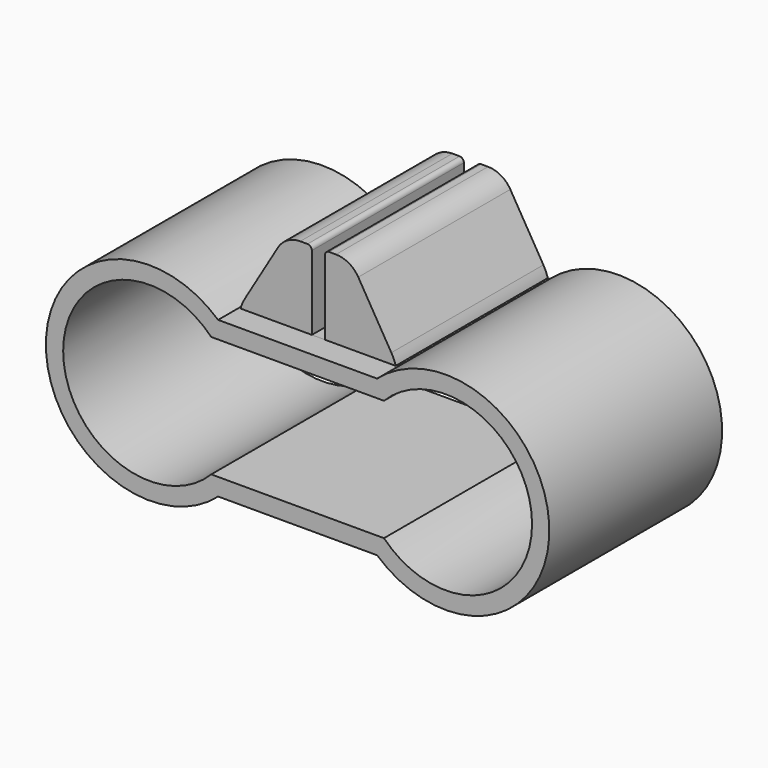
from build123d import *

# Parameters (mm, degrees)
F2_DEPTH = 25
F4_DEPTH = 22
F5_R     = 5
F6_R     = 0.5
F7_SIZE  = 0.5


# Not quite as in the source:
# - a feature of the source that left no trace in its solid (it failed there, or was rolled back) is left out


with BuildPart() as f2:
    # F1 (on Front) → F2 (new body)
    with BuildSketch(Plane.XZ):
        with BuildLine():
            Line((-0.75, 9), (-9.2, 9))
            ThreePointArc((-9.2, 9), (-29.1372539332, 0), (-9.2, -9))
            Line((-9.2, -9), (9.2, -9))
            ThreePointArc((9.2, -9), (29.1372539332, 0), (9.2, 9))
            Line((9.2, 9), (9.15, 9))
            Line((9.15, 9), (0.75, 9))
            Line((0.75, 9), (-0.75, 9))
        make_face()
        with BuildLine():
            Line((9.9958255047, -7), (-9.9958255047, -7))
            ThreePointArc((-9.9958255047, -7), (-27.1372539332, 0), (-9.9958255047, 7))
            Line((-9.9958255047, 7), (9.9958255047, 7))
            ThreePointArc((9.9958255047, 7), (27.1372539332, 0), (9.9958255047, -7))
        make_face(mode=Mode.SUBTRACT)
    extrude(amount=F2_DEPTH)


with BuildPart() as f4:
    # F3 (on Front) → F4 (new body)
    with BuildSketch(Plane.XZ):
        with BuildLine():
            Line((-0.75, 18.1), (-2.0917842475, 18.1))
            ThreePointArc((-2.0917842475, 18.1), (-3.576222945, 17.7069986101), (-4.6717373284, 16.6309611689))
            Line((-4.6717373284, 16.6309611689), (-9.2, 9))
            Line((-9.2, 9), (-9.2, 6))
            Line((-9.2, 6), (9.15, 6))
            Line((9.15, 6), (9.15, 9))
            Line((9.15, 9), (4.6217373284, 16.6309611689))
            ThreePointArc((4.6217373284, 16.6309611689), (3.526222945, 17.7069986101), (2.0417842475, 18.1))
            Line((2.0417842475, 18.1), (0.75, 18.1))
            Line((0.75, 18.1), (0.75, 9))
            Line((0.75, 9), (-0.75, 9))
            Line((-0.75, 9), (-0.75, 18.1))
        make_face()
    extrude(amount=F4_DEPTH)

    # F5
    f5_edges = [f4.edges().sort_by_distance(p)[0] for p in [
        (9.15, -11, 9),
        (-9.2, -11, 9),
    ]]
    fillet(f5_edges, radius=F5_R)

    # F6
    f6_edges = [f4.edges().sort_by_distance(p)[0] for p in [
        (-0.75, -11, 18.1),
        (0.75, -11, 18.1),
    ]]
    fillet(f6_edges, radius=F6_R)

    # F7
    f7_edges = [f4.edges().sort_by_distance(p)[0] for p in [
        (-9.2, -11, 6),
        (9.15, -11, 6),
        (-0.025, 0, 6),
        (-0.025, -22, 6),
    ]]
    chamfer(f7_edges, length=F7_SIZE)


solid = Compound([f2.part, f4.part])
